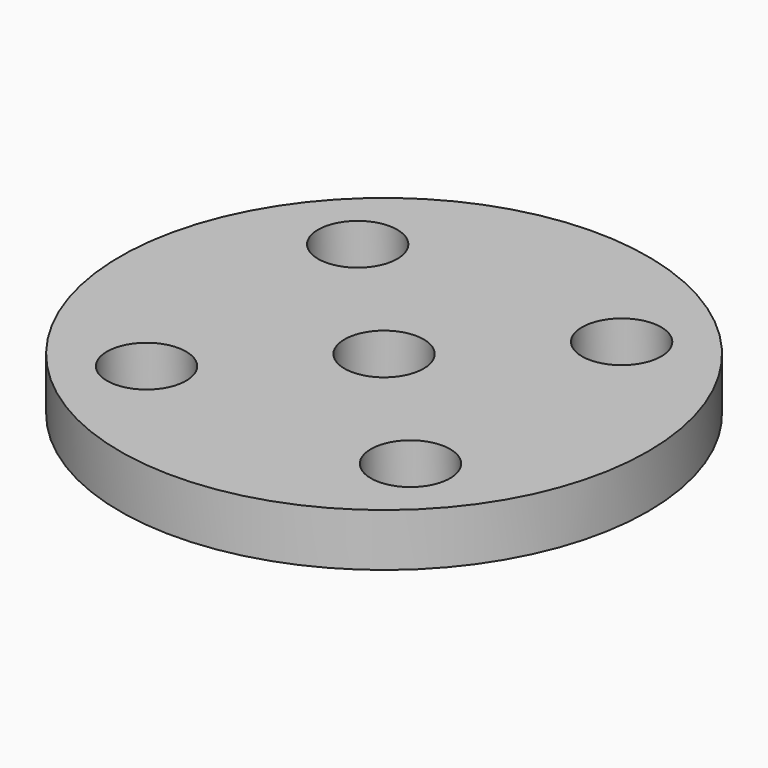
from build123d import *

# Parameters (mm, degrees)
F0_R     = 10
F0_R_2   = 1.5
F1_DEPTH = 2
F3_D     = 3
F4_R     = 4
F4_R_2   = 2.5
F5_DEPTH = 3


# Not quite as in the source:
# - a feature names something its author has since deleted; it is built from what else it names


with BuildPart() as f1:
    # F0 (on Top) → F1 (new body)
    with BuildSketch(Plane.XY):
        Circle(F0_R)
        Circle(F0_R_2, mode=Mode.SUBTRACT)
    extrude(amount=F1_DEPTH)

    # F3 (through all)
    with Locations(Plane.XY.offset(2)):
        with Locations((-5, 5), (5, 5), (5, -5), (-5, -5)):
            Hole(F3_D / 2)

    # F4 (on face) → F5 (join)
    with BuildSketch(Plane(origin=(0, 0, 0), x_dir=(1, 0, 0), z_dir=(0, 0, -1))):
        Circle(F4_R)
        Circle(F4_R_2, mode=Mode.SUBTRACT)
    extrude(amount=F5_DEPTH)


solid = f1.part
